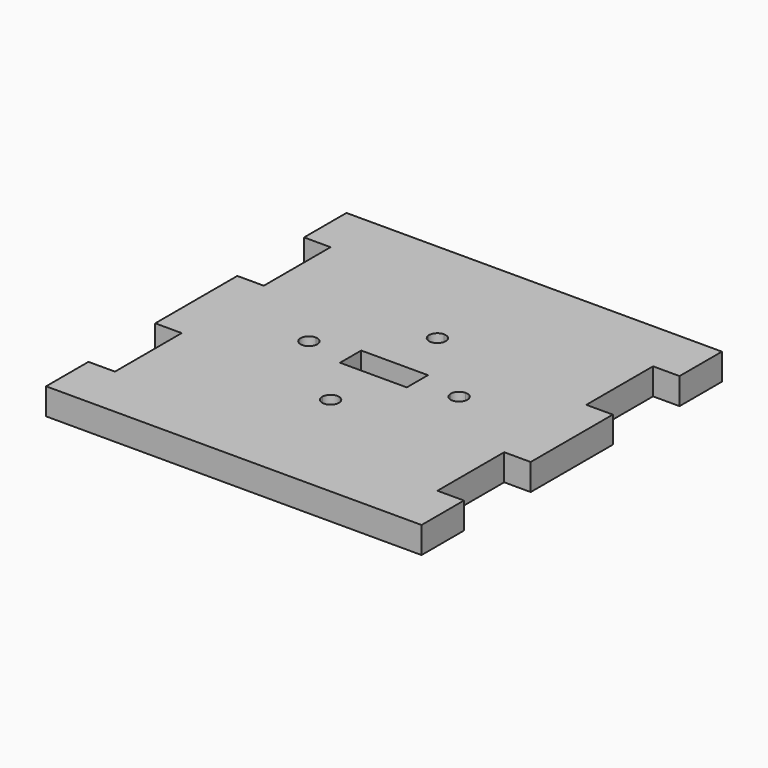
from build123d import *

# Parameters (mm, degrees)
F0_W     = 8
F0_H     = 3.175
F1_DEPTH = 3.175


# Not quite as in the source:
# - a length typed as a fraction of an inch, garbled in the dataset ("3 / 203.2 mm" for 3/8 in), is restored
# - a feature names something its author has since deleted; it is built from what else it names


with BuildPart() as f1:
    # F0 (on Top) → F1 (new body)
    with BuildSketch(Plane.XY):
        Polygon((-19.325, 11.15), (19.325, 11.15), (19.325, 16.15), (22.5, 16.15), (22.5, 22.5), (-22.5, 22.5), (-22.5, 16.15), (-19.325, 16.15), align=None)
        Polygon((-19.325, -11.15), (19.325, -11.15), (19.325, -6.15), (22.5, -6.15), (22.5, 6.15), (19.325, 6.15), (19.325, 11.15), (-19.325, 11.15), (-19.325, 6.15), (-22.5, 6.15), (-22.5, -6.15), (-19.325, -6.15), align=None)
        with BuildLine():
            ThreePointArc((-8.9444444444, -0.9984555975), (-10, 0), (-8.9444444444, 0.9984555975))
            ThreePointArc((-8.9444444444, 0.9984555975), (-6.000579123, 6.7076859042), (0, 9))
            ThreePointArc((0, 9), (6.000579123, 6.7076859042), (8.9444444444, 0.9984555975))
            ThreePointArc((8.9444444444, 0.9984555975), (9.6871842709, 0.7264831573), (10, 0))
            ThreePointArc((10, 0), (9.6871842709, -0.7264831573), (8.9444444444, -0.9984555975))
            ThreePointArc((8.9444444444, -0.9984555975), (6.000579123, -6.7076859042), (0, -9))
            ThreePointArc((0, -9), (-6.000579123, -6.7076859042), (-8.9444444444, -0.9984555975))
        make_face(mode=Mode.SUBTRACT)
        Polygon((-22.5, -22.5), (22.5, -22.5), (22.5, -16.15), (19.325, -16.15), (19.325, -11.15), (-19.325, -11.15), (-19.325, -16.15), (-22.5, -16.15), align=None)
        with BuildLine():
            ThreePointArc((-0.9980449639, 7.9375), (-5.9993482859, 5.2922415047), (-8, 0))
            ThreePointArc((-8, 0), (-5.9993482859, -5.2922415047), (-0.9980449639, -7.9375))
            ThreePointArc((-0.9980449639, -7.9375), (0, -7), (0.9980449639, -7.9375))
            ThreePointArc((0.9980449639, -7.9375), (5.9993482859, -5.2922415047), (8, 0))
            ThreePointArc((8, 0), (5.9993482859, 5.2922415047), (0.9980449639, 7.9375))
            ThreePointArc((0.9980449639, 7.9375), (0, 7), (-0.9980449639, 7.9375))
        make_face()
        Rectangle(F0_W, F0_H, mode=Mode.SUBTRACT)
        with BuildLine():
            ThreePointArc((-8.9444444444, 0.9984555975), (-8.2735168427, 0.6871842709), (-8, 0))
            ThreePointArc((-8, 0), (-5.9993482859, 5.2922415047), (-0.9980449639, 7.9375))
            ThreePointArc((-0.9980449639, 7.9375), (-0.7288689869, 8.6846531969), (0, 9))
            ThreePointArc((0, 9), (-6.000579123, 6.7076859042), (-8.9444444444, 0.9984555975))
        make_face()
        with BuildLine():
            ThreePointArc((8.9444444444, 0.9984555975), (6.000579123, 6.7076859042), (0, 9))
            ThreePointArc((0, 9), (0.7071067812, 8.7071067812), (1, 8))
            ThreePointArc((1, 8), (0.9995111215, 7.9687347151), (0.9980449639, 7.9375))
            ThreePointArc((0.9980449639, 7.9375), (5.9993482859, 5.2922415047), (8, 0))
            ThreePointArc((8, 0), (8.2735168427, 0.6871842709), (8.9444444444, 0.9984555975))
        make_face()
        with BuildLine():
            ThreePointArc((1, -8), (0.7071067812, -8.7071067812), (0, -9))
            ThreePointArc((0, -9), (6.000579123, -6.7076859042), (8.9444444444, -0.9984555975))
            ThreePointArc((8.9444444444, -0.9984555975), (8.2735168427, -0.6871842709), (8, 0))
            ThreePointArc((8, 0), (5.9993482859, -5.2922415047), (0.9980449639, -7.9375))
            ThreePointArc((0.9980449639, -7.9375), (0.9995111215, -7.9687347151), (1, -8))
        make_face()
        with BuildLine():
            ThreePointArc((-0.9980449639, -7.9375), (-5.9993482859, -5.2922415047), (-8, 0))
            ThreePointArc((-8, 0), (-8.2735168427, -0.6871842709), (-8.9444444444, -0.9984555975))
            ThreePointArc((-8.9444444444, -0.9984555975), (-6.000579123, -6.7076859042), (0, -9))
            ThreePointArc((0, -9), (-0.7288689869, -8.6846531969), (-0.9980449639, -7.9375))
        make_face()
    extrude(amount=F1_DEPTH)


solid = f1.part
